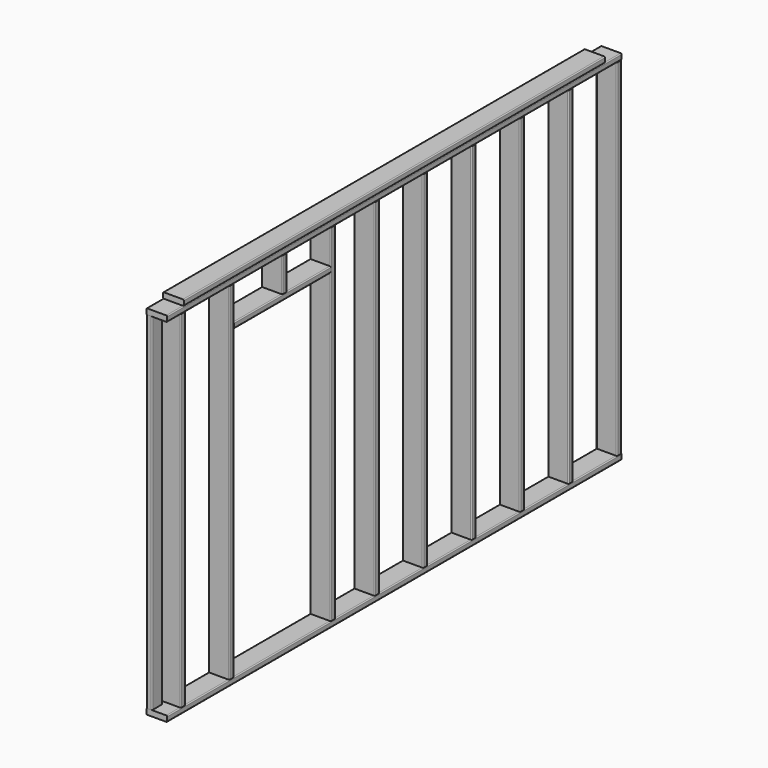
from build123d import *

# Parameters (mm, degrees)
F0_W      = 150
F0_H      = 1.5
F1_DEPTH  = 5.5
F2_W      = 1.5
F2_H      = 91.5
F3_DEPTH  = 5.5
F4_W      = 32
F4_H      = 1.5
F5_DEPTH  = 5.5
F6_W      = 139
F6_H      = 1.5
F6_W_2    = 1.5
F6_H_2    = 9
F7_DEPTH  = 5.5
F8_R      = 0.25
F8_2_R    = 0.25
F8_3_R    = 0.25
F8_4_R    = 0.25
F8_5_R    = 0.25
F8_6_R    = 0.25
F8_7_R    = 0.25
F8_8_R    = 0.25
F8_9_R    = 0.25
F8_10_R   = 0.25
F8_11_R   = 0.25
F8_12_R   = 0.25
F9_W      = 3.5
F9_H      = 91.5
F10_DEPTH = 1.5
F11_R     = 0.25


# Not quite as in the source:
# - a feature names something its author has since deleted; it is built from what else it names


with BuildPart() as f1:
    # F0 (on Right) → F1 (new body)
    with BuildSketch(Plane.YZ):
        with Locations((9.6768632531, -17.3856742978)):
            Rectangle(F0_W, F0_H)
    extrude(amount=F1_DEPTH)

    # F8#12
    f8_12_edges = [f1.edges().sort_by_distance(p)[0] for p in [
        (0, 9.676863, -18.135674),
        (0, 9.676863, -16.635674),
        (5.5, 9.676863, -16.635674),
        (5.5, 9.676863, -18.135674),
    ]]
    fillet(f8_12_edges, radius=F8_12_R)


with BuildPart() as f3:
    # F2 (on Right) → F3 (new body)
    with BuildSketch(Plane.YZ):
        with Locations((83.9268632531, 29.1143257022)):
            Rectangle(F2_W, F2_H)
    extrude(amount=F3_DEPTH)

    # F8#6
    f8_6_edges = [f3.edges().sort_by_distance(p)[0] for p in [
        (5.5, 84.676863, 29.114326),
        (0, 84.676863, 29.114326),
        (0, 83.176863, 29.114326),
        (5.5, 83.176863, 29.114326),
    ]]
    fillet(f8_6_edges, radius=F8_6_R)


with BuildPart() as f3b:
    # F2 (on Right) → F3, piece 2 (new body)
    with BuildSketch(Plane.YZ):
        with Locations((67.9268632531, 29.1143257022)):
            Rectangle(F2_W, F2_H)
    extrude(amount=F3_DEPTH)

    # F8#3
    f8_3_edges = [f3b.edges().sort_by_distance(p)[0] for p in [
        (0, 67.176863, 29.114326),
        (0, 68.676863, 29.114326),
        (5.5, 68.676863, 29.114326),
        (5.5, 67.176863, 29.114326),
    ]]
    fillet(f8_3_edges, radius=F8_3_R)


with BuildPart() as f3c:
    # F2 (on Right) → F3, piece 3 (new body)
    with BuildSketch(Plane.YZ):
        with Locations((51.9268632531, 29.1143257022)):
            Rectangle(F2_W, F2_H)
    extrude(amount=F3_DEPTH)

    # F8#5
    f8_5_edges = [f3c.edges().sort_by_distance(p)[0] for p in [
        (0, 51.176863, 29.114326),
        (5.5, 52.676863, 29.114326),
        (0, 52.676863, 29.114326),
        (5.5, 51.176863, 29.114326),
    ]]
    fillet(f8_5_edges, radius=F8_5_R)


with BuildPart() as f3d:
    # F2 (on Right) → F3, piece 4 (new body)
    with BuildSketch(Plane.YZ):
        with Locations((35.9268632531, 29.1143257022)):
            Rectangle(F2_W, F2_H)
    extrude(amount=F3_DEPTH)

    # F8#4
    f8_4_edges = [f3d.edges().sort_by_distance(p)[0] for p in [
        (0, 35.176863, 29.114326),
        (5.5, 36.676863, 29.114326),
        (0, 36.676863, 29.114326),
        (5.5, 35.176863, 29.114326),
    ]]
    fillet(f8_4_edges, radius=F8_4_R)


with BuildPart() as f3e:
    # F2 (on Right) → F3, piece 5 (new body)
    with BuildSketch(Plane.YZ):
        with Locations((19.9268632531, 29.1143257022)):
            Rectangle(F2_W, F2_H)
    extrude(amount=F3_DEPTH)

    # F8
    f8_edges = [f3e.edges().sort_by_distance(p)[0] for p in [
        (0, 20.676863, 29.114326),
        (5.5, 20.676863, 29.114326),
        (0, 19.176863, 29.114326),
        (5.5, 19.176863, 29.114326),
    ]]
    fillet(f8_edges, radius=F8_R)


with BuildPart() as f3f:
    # F2 (on Right) → F3, piece 6 (new body)
    with BuildSketch(Plane.YZ):
        with Locations((3.9268632531, 29.1143257022)):
            Rectangle(F2_W, F2_H)
    extrude(amount=F3_DEPTH)

    # F8#2
    f8_2_edges = [f3f.edges().sort_by_distance(p)[0] for p in [
        (0, 3.176863, 29.114326),
        (5.5, 4.676863, 29.114326),
        (5.5, 3.176863, 29.114326),
        (0, 4.676863, 29.114326),
    ]]
    fillet(f8_2_edges, radius=F8_2_R)


with BuildPart() as f3g:
    # F2 (on Right) → F3, piece 7 (new body)
    with BuildSketch(Plane.YZ):
        with Locations((-10.5731367469, 29.1143257022)):
            Rectangle(F2_W, F2_H)
    extrude(amount=F3_DEPTH)

    # F8#9
    f8_9_edges = [f3g.edges().sort_by_distance(p)[0] for p in [
        (5.5, -11.323137, 29.114326),
        (0, -9.823137, 29.114326),
        (5.5, -9.823137, 29.114326),
        (0, -11.323137, 29.114326),
    ]]
    fillet(f8_9_edges, radius=F8_9_R)


with BuildPart() as f3h:
    # F2 (on Right) → F3, piece 8 (new body)
    with BuildSketch(Plane.YZ):
        with Locations((-44.0731367469, 29.1143257022)):
            Rectangle(F2_W, F2_H)
    extrude(amount=F3_DEPTH)

    # F8#7
    f8_7_edges = [f3h.edges().sort_by_distance(p)[0] for p in [
        (5.5, -43.323137, 29.114326),
        (0, -44.823137, 29.114326),
        (0, -43.323137, 29.114326),
        (5.5, -44.823137, 29.114326),
    ]]
    fillet(f8_7_edges, radius=F8_7_R)


with BuildPart() as f3i:
    # F2 (on Right) → F3, piece 9 (new body)
    with BuildSketch(Plane.YZ):
        with Locations((-60.0731367469, 29.1143257022)):
            Rectangle(F2_W, F2_H)
    extrude(amount=F3_DEPTH)

    # F8#8
    f8_8_edges = [f3i.edges().sort_by_distance(p)[0] for p in [
        (0, -59.323137, 29.114326),
        (5.5, -60.823137, 29.114326),
        (0, -60.823137, 29.114326),
        (5.5, -59.323137, 29.114326),
    ]]
    fillet(f8_8_edges, radius=F8_8_R)


with BuildPart() as f5:
    # F4 (on Right) → F5 (new body)
    with BuildSketch(Plane.YZ):
        Polygon((-65.3231367469, 74.8643257022), (84.6768632531, 74.8643257022), (84.6768632531, 76.3643257022), (79.1768632531, 76.3643257022), (-59.8231367469, 76.3643257022), (-65.3231367469, 76.3643257022), align=None)
        with Locations((-27.3231367469, 65.1143257022)):
            Rectangle(F4_W, F4_H)
    extrude(amount=F5_DEPTH)

    # F8#10
    f8_10_edges = [f5.edges().sort_by_distance(p)[0] for p in [
        (5.5, -27.323137, 65.864326),
        (0, -27.323137, 64.364326),
        (5.5, -27.323137, 64.364326),
        (0, -27.323137, 65.864326),
        (5.5, 9.676863, 74.864326),
        (0, 9.676863, 76.364326),
        (5.5, 9.676863, 76.364326),
        (0, 9.676863, 74.864326),
    ]]
    fillet(f8_10_edges, radius=F8_10_R)


with BuildPart() as f7:
    # F6 (on Right) → F7 (new body)
    with BuildSketch(Plane.YZ):
        with Locations((9.6768632531, 77.1143257022)):
            Rectangle(F6_W, F6_H)
        with Locations((-26.5731367469, 70.3643257022)):
            Rectangle(F6_W_2, F6_H_2)
    extrude(amount=F7_DEPTH)

    # F8#11
    f8_11_edges = [f7.edges().sort_by_distance(p)[0] for p in [
        (0, 9.676863, 77.864326),
        (5.5, 9.676863, 77.864326),
        (0, 9.676863, 76.364326),
        (5.5, 9.676863, 76.364326),
        (5.5, -25.823137, 70.364326),
        (5.5, -27.323137, 70.364326),
        (0, -27.323137, 70.364326),
        (0, -25.823137, 70.364326),
    ]]
    fillet(f8_11_edges, radius=F8_11_R)


with BuildPart() as f10:
    # F9 (on Right) → F10 (new body)
    with BuildSketch(Plane.YZ):
        with Locations((-63.5731367469, 29.1143257022)):
            Rectangle(F9_W, F9_H)
    extrude(amount=F10_DEPTH)

    # F11
    f11_edges = [f10.edges().sort_by_distance(p)[0] for p in [
        (0, -61.823137, 29.114326),
        (0, -65.323137, 29.114326),
        (1.5, -61.823137, 29.114326),
        (1.5, -65.323137, 29.114326),
    ]]
    fillet(f11_edges, radius=F11_R)


solid = Compound([f1.part, f3.part, f3b.part, f3c.part, f3d.part, f3e.part, f3f.part, f3g.part, f3h.part, f3i.part, f5.part, f7.part, f10.part])
